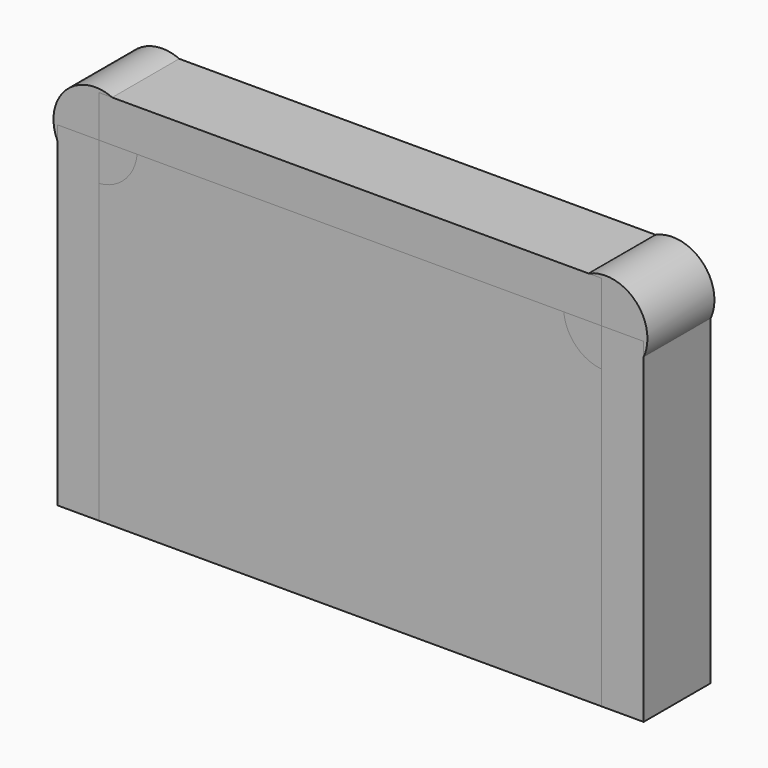
from build123d import *

# Parameters (mm, degrees)
F0_W     = 76.2
F0_H     = 50.8
F3_DEPTH = 12.7
F1_R     = 6.35
F2_W     = 6.35
F2_H     = 50.8
F2_W_2   = 76.2
F2_H_2   = 6.35


# Not quite as in the source:
# - a feature of the source that left no trace in its solid (it failed there, or was rolled back) is left out


with BuildPart() as f3:
    # F0 (on Front) → F3 (new body)
    with BuildSketch(Plane.XZ):
        Rectangle(F0_W, F0_H)
    extrude(amount=F3_DEPTH)


with BuildPart() as f3b:
    # F1 (on Front) → F3, piece 2 (new body)
    with BuildSketch(Plane.XZ):
        with Locations((-38.6804193258, 25.9450823069)):
            Circle(F1_R)
    extrude(amount=F3_DEPTH)


with BuildPart() as f3c:
    # F1 (on Front) → F3, piece 3 (new body)
    with BuildSketch(Plane.XZ):
        with Locations((38.6804193258, 25.9450823069)):
            Circle(F1_R)
    extrude(amount=F3_DEPTH)


with BuildPart() as f3d:
    # F2 (on Front) → F3, piece 4 (new body)
    with BuildSketch(Plane.XZ):
        with Locations((41.275, 0)):
            Rectangle(F2_W, F2_H)
    extrude(amount=F3_DEPTH)


with BuildPart() as f3e:
    # F2 (on Front) → F3, piece 5 (new body)
    with BuildSketch(Plane.XZ):
        with Locations((0, 28.575)):
            Rectangle(F2_W_2, F2_H_2)
    extrude(amount=F3_DEPTH)


with BuildPart() as f3f:
    # F2 (on Front) → F3, piece 6 (new body)
    with BuildSketch(Plane.XZ):
        with Locations((-41.275, 0)):
            Rectangle(F2_W, F2_H)
    extrude(amount=F3_DEPTH)


solid = Compound([f3.part, f3b.part, f3c.part, f3d.part, f3e.part, f3f.part])
